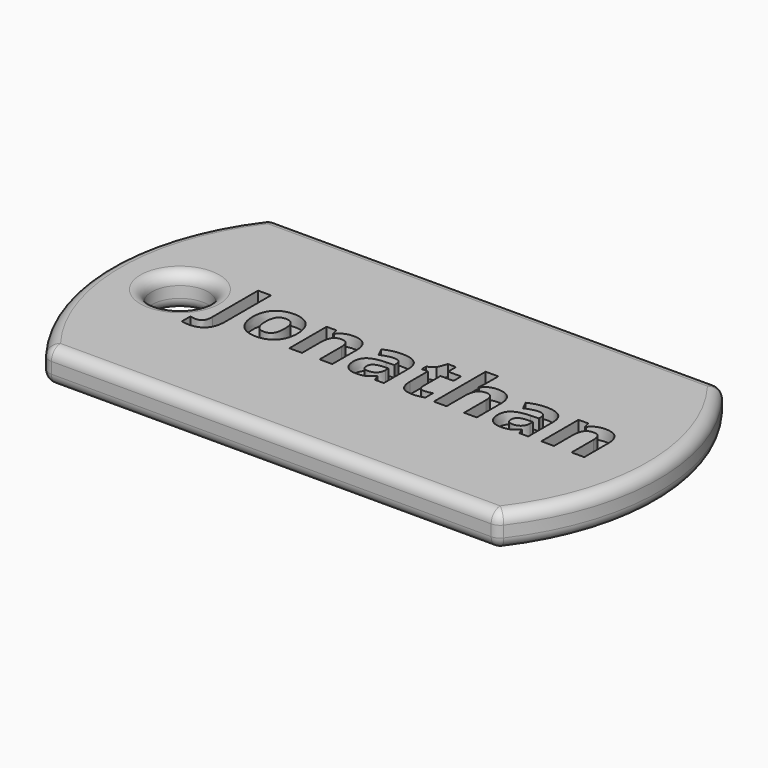
from build123d import *

# Parameters (mm, degrees)
F0_R         = 2.5
F1_DEPTH     = 3
F2_TEXT_SIZE = 7.5627131233
F3_DEPTH     = 1
F4_TEXT_SIZE = 23.1166150671
F5_DEPTH     = 1
F6_R         = 1


# Not quite as in the source:
# - Text() gives the source's letters only with a copy of the font that has no kerning and outlines rounded to 1/6400 em; it was checked with that copy


with BuildPart() as f1:
    # F0 (on Top) → F1 (new body)
    with BuildSketch(Plane.XY):
        with BuildLine():
            Line((20, 12.5), (-20, 12.5))
            ThreePointArc((-20, 12.5), (-24.387505004, 0), (-20, -12.5))
            Line((-20, -12.5), (20, -12.5))
            ThreePointArc((20, -12.5), (24.387505004, 0), (20, 12.5))
        make_face()
        with Locations((-18.112494996, 0)):
            Circle(F0_R, mode=Mode.SUBTRACT)
    extrude(amount=F1_DEPTH)

    # F2 (on face) → F3 (cut)
    with BuildSketch(Plane.XY.offset(3)):
        with Locations((-14.4549424787, -2.1526622553)):
            Text('Jonathan', F2_TEXT_SIZE, font='Open Sans', font_style=FontStyle.BOLD, text_align=(TextAlign.LEFT, TextAlign.BOTTOM))
    extrude(amount=-F3_DEPTH, mode=Mode.SUBTRACT)

    # F4 (on face) → F5 (cut)
    with BuildSketch(Plane(origin=(0, 0, 0), x_dir=(1, 0, 0), z_dir=(0, 0, -1))):
        with Locations((-13.4898121623, -8.2049270891)):
            Text('Liu', F4_TEXT_SIZE, font='Open Sans', font_style=FontStyle.BOLD, text_align=(TextAlign.LEFT, TextAlign.BOTTOM))
    extrude(amount=-F5_DEPTH, mode=Mode.SUBTRACT)

    # F6
    f6_edges = [f1.edges().sort_by_distance(p)[0] for p in [
        (20, -12.5, 1.5),
        (20, 12.5, 1.5),
        (24.387505, 0, 0),
        (24.387505, 0, 3),
        (-20, -12.5, 1.5),
        (0, -12.5, 0),
        (0, -12.5, 3),
        (-15.612495, 0, 1.5),
        (-20.612495, 0, 0),
        (-20.612495, 0, 3),
        (-20, 12.5, 1.5),
        (-24.387505, 0, 0),
        (-24.387505, 0, 3),
        (0, 12.5, 0),
        (0, 12.5, 3),
    ]]
    fillet(f6_edges, radius=F6_R)


solid = f1.part
